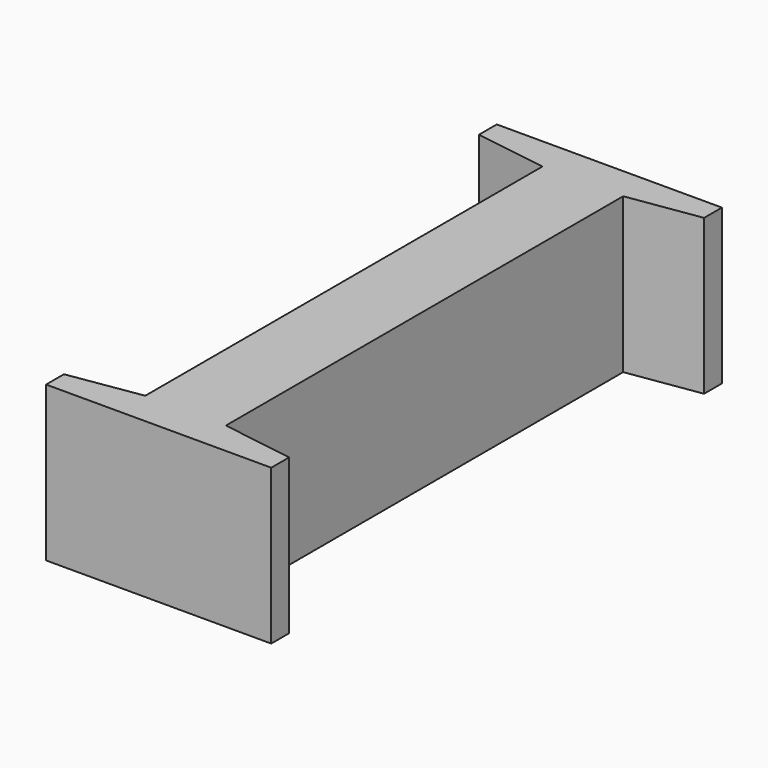
from build123d import *

# Parameters (mm, degrees)
F0_TEXT_SIZE = 141.1111111111
F1_DEPTH     = 25.4


# Not quite as in the source:
# - Text() gives the source's letters only with a copy of the font that has no kerning and outlines rounded to 1/6400 em; it was checked with that copy


with BuildPart() as f1:
    # F0 (on Top) → F1 (new body)
    with BuildSketch(Plane.XY):
        with Locations((-25.9094512032, -58.2234964548)):
            Text('I', F0_TEXT_SIZE, font='Tinos', text_align=(TextAlign.LEFT, TextAlign.BOTTOM))
    extrude(amount=F1_DEPTH)


solid = f1.part
